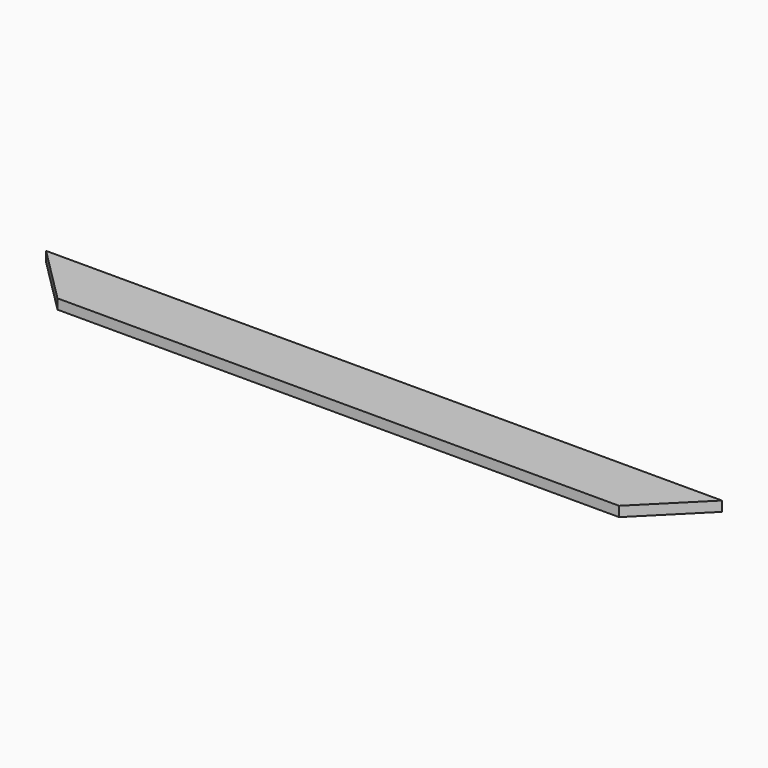
from build123d import *

# Parameters (mm, degrees)
F0_W     = 1420
F0_H     = 120
F1_DEPTH = 21
F2_SIZE  = 119.99999


# Not quite as in the source:
# - a fillet or chamfer is up to 0.001 mm smaller than in the source, because OpenCascade refuses the exact size


with BuildPart() as f1:
    # F0 (on Top) → F1 (new body)
    with BuildSketch(Plane.XY):
        Rectangle(F0_W, F0_H)
    extrude(amount=F1_DEPTH)

    # F2 (size 120 in the source; OpenCascade refuses exactly that, so slightly less here)
    f2_edges = [f1.edges().sort_by_distance(p)[0] for p in [
        (-710, -60, 10.5),
        (710, -60, 10.5),
    ]]
    chamfer(f2_edges, length=F2_SIZE)


solid = f1.part
